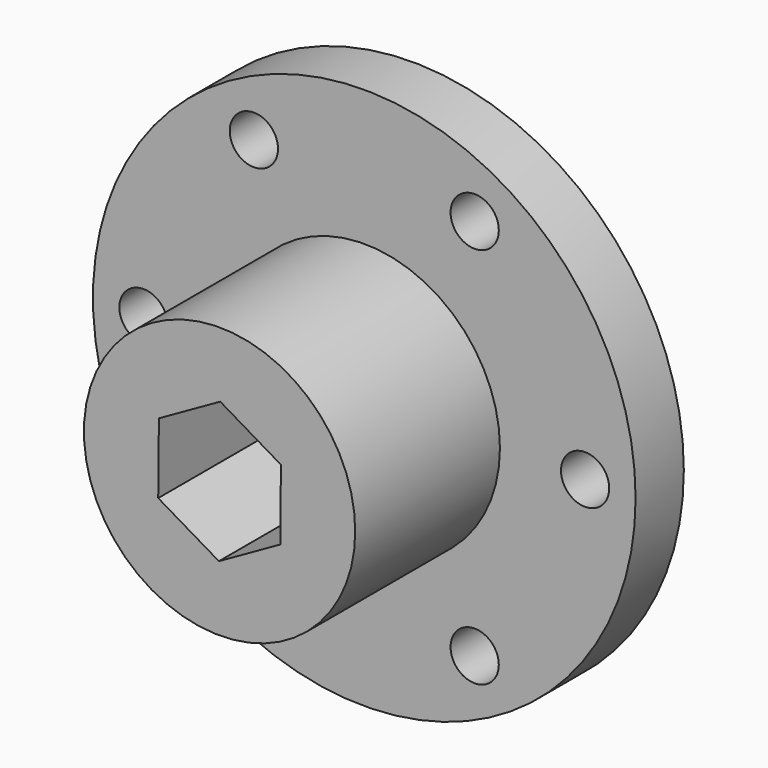
from build123d import *

# Parameters (mm, degrees)
F0_R     = 14.2875
F1_DEPTH = 25.4
F0_R_2   = 28.575
F0_R_3   = 2.54
F2_DEPTH = 6.35


# Not quite as in the source:
# - the program builds the solid bodies; features that only make, move or delete a surface that nothing else refers to are left out


with BuildPart() as f1:
    # F0 (on Front) → F1 (new body)
    with BuildSketch(Plane.XZ):
        Circle(F0_R)
        Polygon((-6.4620758334, -3.6480295337), (-6.3903241666, 3.772307066), (0.0717516667, 7.4203365997), (6.4620758334, 3.6480295337), (6.3903241666, -3.772307066), (-0.0717516667, -7.4203365997), align=None, mode=Mode.SUBTRACT)
    extrude(amount=F1_DEPTH)


with BuildPart() as f2:
    # F0 (on Front) → F2 (new body)
    with BuildSketch(Plane.XZ):
        Circle(F0_R_2)
        with Locations((-11.6278267134, -20.1399866492)):
            Circle(F0_R_3, mode=Mode.SUBTRACT)
        with Locations((11.6278267134, -20.1399866492)):
            Circle(F0_R_3, mode=Mode.SUBTRACT)
        with Locations((-23.2556534267, 0)):
            Circle(F0_R_3, mode=Mode.SUBTRACT)
        with Locations((-11.6278267134, 20.1399866492)):
            Circle(F0_R_3, mode=Mode.SUBTRACT)
        Circle(F0_R, mode=Mode.SUBTRACT)
        with Locations((23.2556534267, 0)):
            Circle(F0_R_3, mode=Mode.SUBTRACT)
        with Locations((11.6278267134, 20.1399866492)):
            Circle(F0_R_3, mode=Mode.SUBTRACT)
    extrude(amount=F2_DEPTH)


solid = Compound([f1.part, f2.part])
